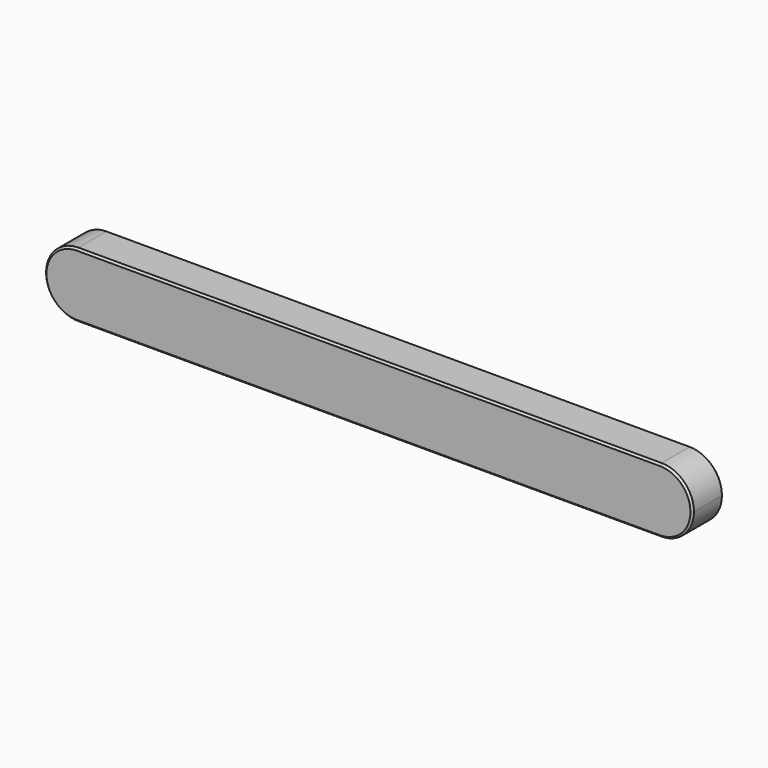
from build123d import *

# Parameters (mm, degrees)
F0_W     = 200
F0_H     = 20
F1_DEPTH = 6
F2_R     = 9.99999
F3_SIZE  = 0.6


# Not quite as in the source:
# - a fillet or chamfer is up to 0.001 mm smaller than in the source, because OpenCascade refuses the exact size


with BuildPart() as f1:
    # F0 (on Front) → F1 (new body, symmetric)
    with BuildSketch(Plane.XZ):
        Rectangle(F0_W, F0_H)
    extrude(amount=F1_DEPTH, both=True)

    # F2 (radius 10 in the source; OpenCascade refuses exactly that, so slightly less here)
    f2_edges = [f1.edges().sort_by_distance(p)[0] for p in [
        (100, 0, -10),
        (100, 0, 10),
        (-100, 0, -10),
        (-100, 0, 10),
    ]]
    fillet(f2_edges, radius=F2_R)

    # F3
    f3_edges = [f1.edges().sort_by_distance(p)[0] for p in [
        (0, -6, 10),
        (100, -6, 0),
        (97.071071, -6, -7.071071),
        (97.071071, -6, 7.071071),
        (0, -6, -10),
        (-97.071071, -6, -7.071071),
        (-97.071071, -6, 7.071071),
        (-100, -6, 0),
        (100, 6, 0),
        (97.071071, 6, -7.071071),
        (97.071071, 6, 7.071071),
        (0, 6, -10),
        (0, 6, 10),
        (-97.071071, 6, -7.071071),
        (-97.071071, 6, 7.071071),
        (-100, 6, 0),
    ]]
    chamfer(f3_edges, length=F3_SIZE)


solid = f1.part
